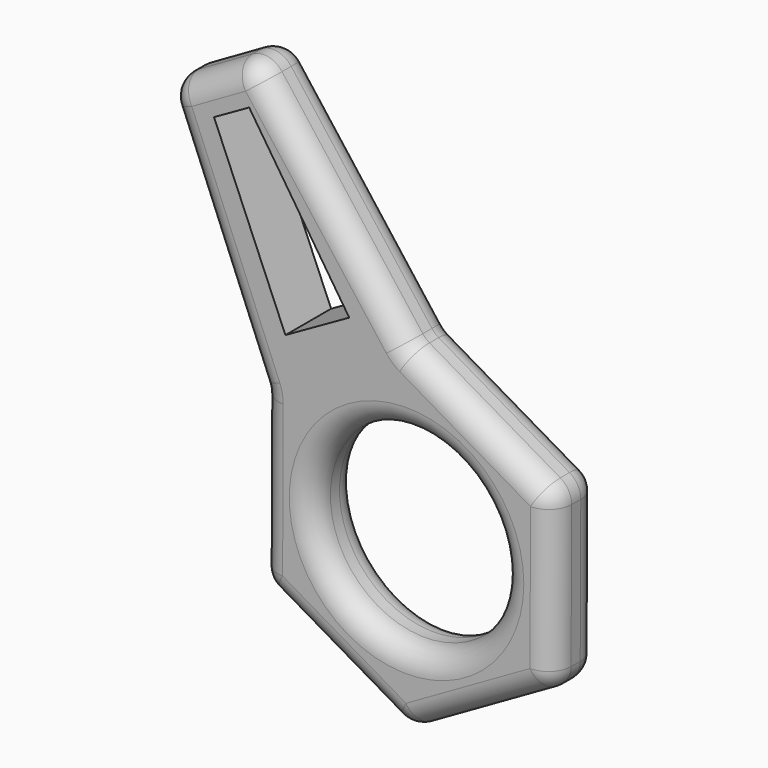
from build123d import *

# Parameters (mm, degrees)
F0_R     = 21.014231477
F1_DEPTH = 12.7
F2_F1_R  = 5.08
F2_F2_R  = 5.08


with BuildPart() as f1:
    # F0 (on Front) → F1 (new body)
    with BuildSketch(Plane.XZ):
        Polygon((-51.5739838451, 57.903360525), (-29.9211297043, 5.0337655893), (2.754318782, 23.7208167973), (-31.8911919502, 69.2358331578), align=None)
        Polygon((-32.4213020707, 59.6586255942), (-10.1648603382, 25.7348876013), (-24.3627145166, 17.7003582495), (-40.2510521891, 55.227790036), align=None, mode=Mode.SUBTRACT)
        Polygon((-29.9211297043, 5.0337655893), (-30.0753928796, -32.6075284839), (2.4457924315, -51.5617713492), (35.1212409178, -32.8747201412), (35.2755040931, 4.766573932), (2.754318782, 23.7208167973), align=None)
        with Locations((2.5902532507, -13.814676553)):
            Circle(F0_R, mode=Mode.SUBTRACT)
    extrude(amount=F1_DEPTH)

    # F2: fillet of radius 5.08 on 22 edges, made by hand

    # F2_f1
    f2_f1_edges = [f1.edges().sort_by_distance(p)[0] for p in [
        (-29.9211297043, -6.35, 5.0337655893),
        (2.754318782, -6.35, 23.7208167973),
    ]]
    fillet(f2_f1_edges, radius=F2_F1_R)

    # F2_f2
    f2_f2_edges = [f1.edges().sort_by_distance(p)[0] for p in [
        (-18.4239782263, -12.7, -13.814676553),
        (-30.0753928796, -6.35, -32.6075284839),
        (-30.0003324711, 0, -14.2922636402),
        (-30.0003324711, -12.7, -14.2922636402),
        (2.4457924315, -6.35, -51.5617713492),
        (-13.8148002241, 0, -42.0846499165),
        (-13.8148002241, -12.7, -42.0846499165),
        (35.1212409178, -6.35, -32.8747201412),
        (18.7835166747, 0, -42.2182457452),
        (18.7835166747, -12.7, -42.2182457452),
        (35.2755040931, -6.35, 4.766573932),
        (35.1983725055, 0, -14.0540731046),
        (35.1983725055, -12.7, -14.0540731046),
        (19.4511663483, 0, 13.9894339824),
        (19.4511663483, -12.7, 13.9894339824),
        (-31.8911919502, -6.35, 69.2358331578),
        (-51.5739838451, -6.35, 57.903360525),
        (-41.7325878977, 0, 63.5695968414),
        (-41.7325878977, -12.7, 63.5695968414),
        (-18.4239782263, 0, -13.814676553),
        (2.8201605652, -12.7, 23.7952939078),
        (2.8201605652, 0, 23.7952939078),
        (-30.0188752401, -12.7, 5.0147331632),
        (-30.0188752401, 0, 5.0147331632),
    ]]
    fillet(f2_f2_edges, radius=F2_F2_R)


solid = f1.part
